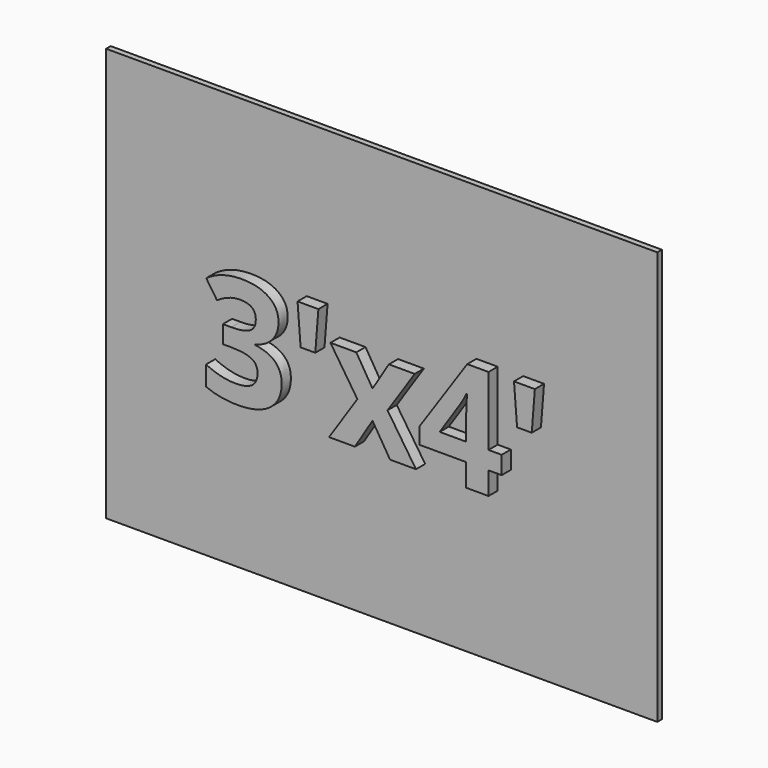
from build123d import *

# Parameters (mm, degrees)
F0_W         = 1219.2
F0_H         = 914.4
F1_DEPTH     = 12.7
F2_TEXT_SIZE = 338.3846794338
F3_DEPTH     = 25.4
F4_TEXT_SIZE = 338.3846794338
F5_DEPTH     = 25.4


# Not quite as in the source:
# - a feature names something its author has since deleted; it is built from what else it names
# - Text() gives the source's letters only with a copy of the font that has no kerning and outlines rounded to 1/6400 em; it was checked with that copy


with BuildPart() as f1:
    # F0 (on Front) → F1 (new body)
    with BuildSketch(Plane.XZ):
        with Locations((609.6, 457.2)):
            Rectangle(F0_W, F0_H)
    extrude(amount=F1_DEPTH)

    # F2 (on face) → F3 (join)
    with BuildSketch(Plane.XZ.offset(12.7)):
        with Locations((228.6, 335.3815154038)):
            Text("3'x4'", F2_TEXT_SIZE, font='Open Sans', font_style=FontStyle.BOLD, text_align=(TextAlign.LEFT, TextAlign.BOTTOM))
    extrude(amount=F3_DEPTH)

    # F4 (on face) → F5 (join)
    with BuildSketch(Plane(origin=(0, 0, 0), x_dir=(-1, 0, 0), z_dir=(0, 1, 0))):
        with Locations((-990.6, 335.3815154038)):
            Text("3'x4'", F4_TEXT_SIZE, font='Open Sans', font_style=FontStyle.BOLD, text_align=(TextAlign.LEFT, TextAlign.BOTTOM))
    extrude(amount=F5_DEPTH)


solid = f1.part
